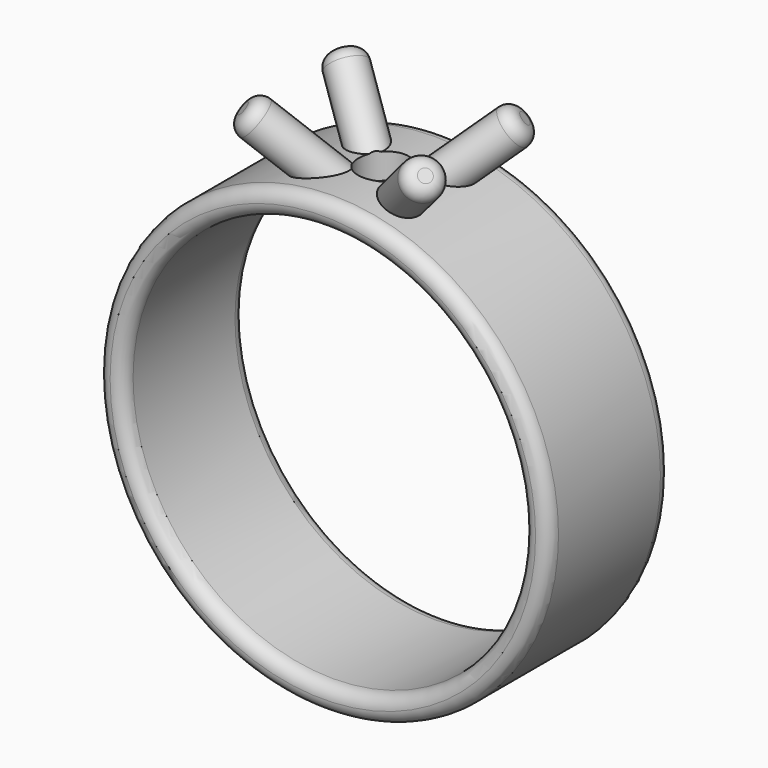
from build123d import *

# Parameters (mm, degrees)
F0_R      = 8.85
F0_R_2    = 7.85
F1_DEPTH  = 3
F10_R     = 0.75
F11_R     = 0.75
F15_R     = 1
F16_DEPTH = 9
F18_R     = 7.85
F19_DEPTH = 25
F20_R     = 0.49999


# Not quite as in the source:
# - a fillet or chamfer is up to 0.001 mm smaller than in the source, because OpenCascade refuses the exact size


with BuildPart() as f1:
    # F0 (on Front) → F1 (new body)
    with BuildSketch(Plane.XZ):
        Circle(F0_R)
        Circle(F0_R_2, mode=Mode.SUBTRACT)
    extrude(amount=F1_DEPTH)

    # F12: sweep along a path in F6
    with BuildLine(Plane(origin=(-3.5442088225, 0, 3.5442088225), x_dir=(0, 1, 0), z_dir=(0.7071067812, 0, -0.7071067812))) as f12_path:
        Line((-0.75, 6.446481747), (-2.440473047, 10.0717128952))
    # F10 (on line) → F12 (sweep)
    with BuildSketch(Plane(origin=(6.5107549732, -4.2935734533, 6.5107549732), x_dir=(0.7676607959, 0.3528089641, -0.5349978853), z_dir=(0.6408563821, -0.4226182617, 0.6408563821))):
        with Locations((-3.8209419121, 3.8345678968)):
            Circle(F10_R)
    sweep(path=f12_path.line)

    # F13: sweep along a path in F7
    with BuildLine(Plane(origin=(3.5442088225, 0, 3.5442088225), x_dir=(0, 1, 0), z_dir=(0.7071067812, 0, 0.7071067812))) as f13_path:
        Line((-0.75, 6.446481747), (-2.440473047, 10.0717128952))
    # F11 (on line) → F13 (sweep)
    with BuildSketch(Plane(origin=(-6.5107549732, -4.2935734533, 6.5107549732), x_dir=(0.2988362387, -0.906307787, -0.2988362387), z_dir=(-0.6408563821, -0.4226182617, 0.6408563821))):
        with Locations((-2.04467007, 5.0122681847)):
            Circle(F11_R)
    sweep(path=f13_path.line)

    # F15 (on offset) → F16 (cut)
    with BuildSketch(Plane.XY.offset(9)):
        Circle(F15_R)
    extrude(amount=-F16_DEPTH, mode=Mode.SUBTRACT)

    # F17: F1 across face


with BuildPart() as f1_1:
    add(f1.part)
    add(f1.part.mirror(Plane(origin=(0, 0, -0.3309567353), x_dir=(1, 0, 0), z_dir=(0, 1, 0))))

    # F18 (on face) → F19 (cut)
    with BuildSketch(Plane.XZ.offset(3)):
        Circle(F18_R)
    extrude(amount=-F19_DEPTH, mode=Mode.SUBTRACT)

    # F20 (radius 0.5 in the source; OpenCascade refuses exactly that, so slightly less here)
    f20_edges = [f1_1.edges().sort_by_distance(p)[0] for p in [
        (-8.85, -3, 0),
        (-7.85, -3, 0),
        (-8.85, 3, 0),
        (-7.85, 3, 0),
        (3.001822, 2.70508, 11.067234),
        (3.001822, -2.70508, 11.067234),
        (-3.801695, -1.760742, 10.890112),
        (-3.801695, 1.760742, 10.890112),
    ]]
    fillet(f20_edges, radius=F20_R)


solid = f1_1.part
